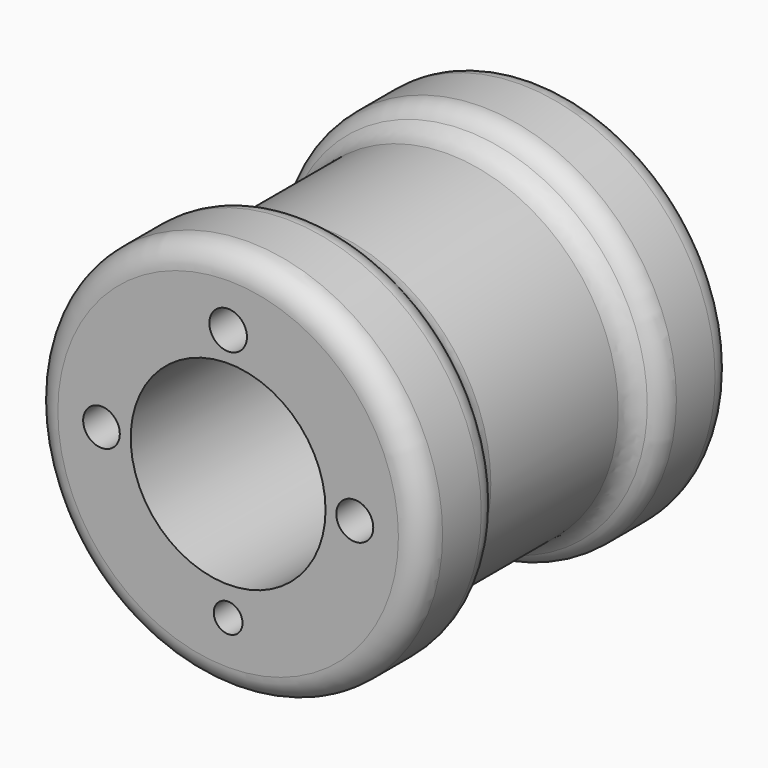
from build123d import *

# Parameters (mm, degrees)
F0_R          = 12.7
F0_R_2        = 6.35
F1_DEPTH      = 25.4
F2_R          = 3.3757627259
F3_DEPTH      = 6.35
F4_R          = 12.7
F4_R_2        = 11.1125
F5_DEPTH      = 12.7
F6_R          = 4.2817922897
F7_DEPTH      = 25.4
F8_R          = 1.2247027219
F8_R_2        = 1.2053090412
F8_R_3        = 0.9363200651
F8_R_4        = 1.1938
F9_DEPTH      = 3.175
F10_S7_R      = 11.1125
F10_T8_DEPTH  = 21
F10_S13_R     = 11.1125
F10_T14_DEPTH = 21
F11_R         = 1.6002


# Not quite as in the source:
# - a fillet or chamfer that OpenCascade refuses, or shapes differently, is made with other operations: its cross-section is extruded or revolved along the edge and cut away or added


with BuildPart() as f1:
    # F0 (on Front) → F1 (new body)
    with BuildSketch(Plane.XZ):
        Circle(F0_R)
        Circle(F0_R_2, mode=Mode.SUBTRACT)
    extrude(amount=F1_DEPTH)

    # F4 (on face) → F5 (cut)
    with BuildSketch(Plane.XZ.offset(6.35)):
        Circle(F4_R)
        Circle(F4_R_2, mode=Mode.SUBTRACT)
    extrude(amount=F5_DEPTH, mode=Mode.SUBTRACT)

    # F8 (on face) → F9 (cut)
    with BuildSketch(Plane.XZ.offset(25.4)):
        with Locations((0, 8.255)):
            Circle(F8_R)
        with Locations((8.255, 0)):
            Circle(F8_R_2)
        with Locations((0, -8.255)):
            Circle(F8_R_3)
        with Locations((-8.255, 0)):
            Circle(F8_R_4)
    extrude(amount=-F9_DEPTH, mode=Mode.SUBTRACT)

    # F10: fillet of radius 1.6002 on 4 edges, made by hand

    # F10_s1 → F10_t2 (revolve, cut)
    with BuildSketch(Plane.XY):
        with BuildLine():
            ThreePointArc((11.0998, -25.4), (12.2313122713, -24.9313122713), (12.7, -23.7998))
            Line((12.7, -23.7998), (12.7, -25.4))
            Line((12.7, -25.4), (11.0998, -25.4))
        make_face()
    revolve(axis=Axis((0, -25.4, 0), (0, -1, 0)), mode=Mode.SUBTRACT)


with BuildPart() as f3:
    # F2 (on Front) → F3 (new body)
    with BuildSketch(Plane.XZ):
        Circle(F2_R)
    extrude(amount=F3_DEPTH)

    # F6 (on face) → F7 (cut)
    with BuildSketch(Plane.XZ.offset(6.35)):
        Circle(F6_R)
    extrude(amount=-F7_DEPTH, mode=Mode.SUBTRACT)


with BuildPart() as f10_tool4:
    # F10_s5 → F10_t6 (revolve)
    with BuildSketch(Plane.XY):
        with BuildLine():
            ThreePointArc((11.0998, -19.05), (12.2313122713, -19.5186877287), (12.7, -20.6502))
            Line((12.7, -20.6502), (12.7, -19.05))
            Line((12.7, -19.05), (11.0998, -19.05))
        make_face()
    revolve(axis=Axis((0, -19.05, 0), (0, -1, 0)))

    # F10_s7 → F10_t8 (cut, symmetric)
    with BuildSketch(Plane.XZ.offset(20.4)):
        Circle(F10_S7_R)
    extrude(amount=F10_T8_DEPTH, both=True, mode=Mode.SUBTRACT)


with BuildPart() as f1_1:
    add(f1.part)

    # F10_t3: cut F10_tool4
    add(f10_tool4.part, mode=Mode.SUBTRACT)


with BuildPart() as f10_tool10:
    # F10_s11 → F10_t12 (revolve)
    with BuildSketch(Plane.XY):
        with BuildLine():
            ThreePointArc((12.7, -4.7498), (12.2313122713, -5.8813122713), (11.0998, -6.35))
            Line((11.0998, -6.35), (12.7, -6.35))
            Line((12.7, -6.35), (12.7, -4.7498))
        make_face()
    revolve(axis=Axis((0, -6.35, 0), (0, -1, 0)))

    # F10_s13 → F10_t14 (cut, symmetric)
    with BuildSketch(Plane.XZ.offset(5.5)):
        Circle(F10_S13_R)
    extrude(amount=F10_T14_DEPTH, both=True, mode=Mode.SUBTRACT)


with BuildPart() as f1_2:
    add(f1_1.part)

    # F10_t9: cut F10_tool10
    add(f10_tool10.part, mode=Mode.SUBTRACT)

    # F10_s15 → F10_t16 (revolve, cut)
    with BuildSketch(Plane.XY):
        with BuildLine():
            ThreePointArc((12.7, -1.6002), (12.2313122713, -0.4686877287), (11.0998, 0))
            Line((11.0998, 0), (12.7, 0))
            Line((12.7, 0), (12.7, -1.6002))
        make_face()
    revolve(axis=Axis((0, 0, 0), (0, -1, 0)), mode=Mode.SUBTRACT)

    # F11
    f11_edges = [f1_2.edges().sort_by_distance(p)[0] for p in [
        (-11.1125, -19.05005, 0),
        (-11.1125, -6.34995, 0),
    ]]
    fillet(f11_edges, radius=F11_R)


solid = f1_2.part
